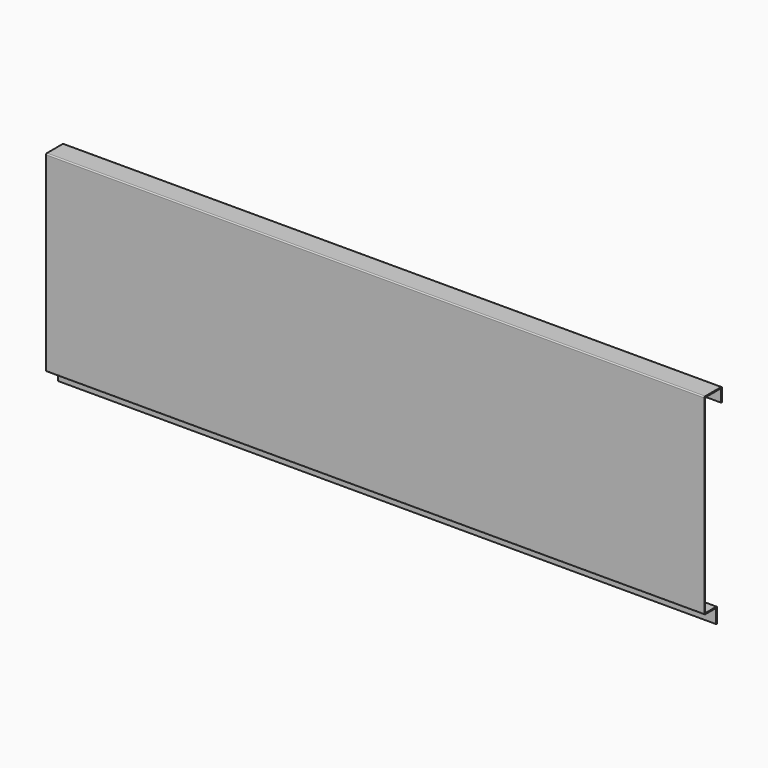
from build123d import *

# Parameters (mm, degrees)
F1_DEPTH = 1200
F2_R     = 2


# Not quite as in the source:
# - a feature names something its author has since deleted; it is built from what else it names


with BuildPart() as f1:
    # F0 (on Right) → F1 (new body)
    with BuildSketch(Plane.YZ):
        Polygon((-18.8378913403, 427.8021101952), (-18.8378913403, 404.8021101952), (-16.8378913403, 404.8021101952), (-16.8378913403, 429.8021101952), (-56.8378913403, 429.8021101952), (-56.8378913403, 79.8021101952), (-29.8378913403, 79.8021101952), (-29.8378913403, 53.8021101952), (-27.8378913403, 53.8021101952), (-27.8378913403, 81.8021101952), (-54.8378913403, 81.8021101952), (-54.8378913403, 427.8021101952), align=None)
    extrude(amount=F1_DEPTH)

    # F2
    f2_edges = [f1.edges().sort_by_distance(p)[0] for p in [
        (600, -56.837891, 429.80211),
        (600, -16.837891, 429.80211),
        (600, -56.837891, 79.80211),
        (600, -27.837891, 81.80211),
        (600, -54.837891, 81.80211),
        (600, -29.837891, 79.80211),
        (600, -18.837891, 427.80211),
        (600, -54.837891, 427.80211),
    ]]
    fillet(f2_edges, radius=F2_R)


solid = f1.part
